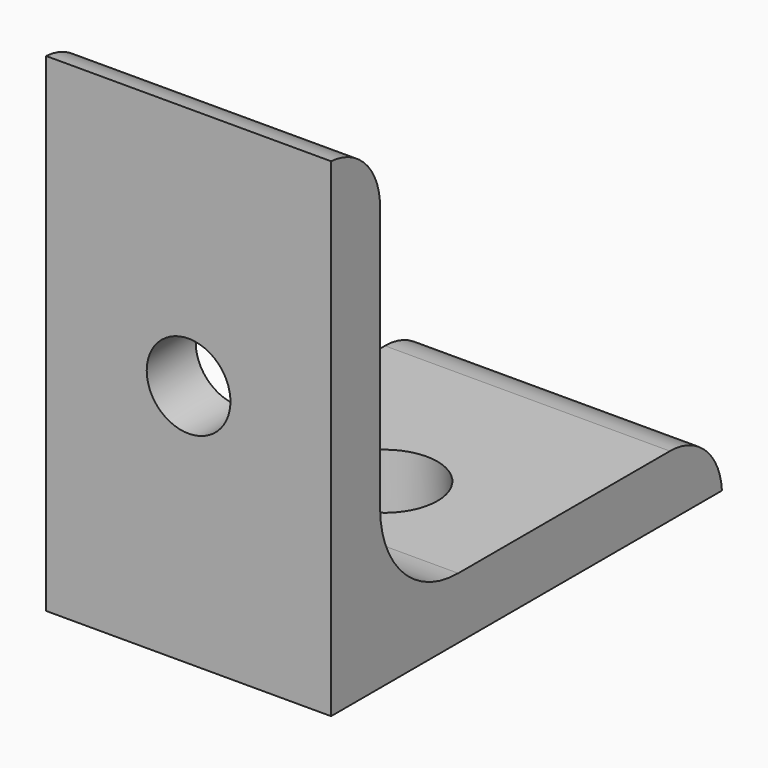
from build123d import *

# Parameters (mm, degrees)
F1_DEPTH    = 22.225
F2_R        = 7.62
F3_T1_DEPTH = 47.5792387778
F4_R        = 3.2639
F5_DEPTH    = 4.7762
F6_R        = 4.1656
F7_DEPTH    = 4.7762


# Not quite as in the source:
# - a fillet or chamfer that OpenCascade refuses, or shapes differently, is made with other operations: its cross-section is extruded or revolved along the edge and cut away or added


with BuildPart() as f1:
    # F0 (on Right) → F1 (new body)
    with BuildSketch(Plane.YZ):
        Polygon((0, 38.1), (0, 0), (38.1, 0), (38.1, 4.7752), (4.7752, 4.7752), (4.7752, 38.1), align=None)
    extrude(amount=-F1_DEPTH)

    # F2
    f2_edges = [f1.edges().sort_by_distance(p)[0] for p in [
        (-11.1125, 4.7752, 4.7752),
    ]]
    fillet(f2_edges, radius=F2_R)

    # F3: fillet of radius 5.08 on 2 edges, made by hand

    # F3_s2 → F3_t1 (cut)
    with BuildSketch(Plane.YZ.offset(-34.9021193889)):
        with BuildLine():
            ThreePointArc((4.7752, 33.0291522444), (3.3934958238, 36.5118247815), (0, 38.1))
            Line((0, 38.1), (4.7752, 38.1))
            Line((4.7752, 38.1), (4.7752, 33.0291522444))
        make_face()
        with BuildLine():
            ThreePointArc((33.0291522444, 4.7752), (36.5118247815, 3.3934958238), (38.1, 0))
            Line((38.1, 0), (38.1, 4.7752))
            Line((38.1, 4.7752), (33.0291522444, 4.7752))
        make_face()
    extrude(amount=F3_T1_DEPTH, mode=Mode.SUBTRACT)

    # F4 (on face) → F5 (cut, through all)
    with BuildSketch(Plane(origin=(0, 4.7752, 0), x_dir=(-1, 0, 0), z_dir=(0, 1, 0))):
        with Locations((11.1125, 19.05)):
            Circle(F4_R)
    extrude(amount=-F5_DEPTH, mode=Mode.SUBTRACT)

    # F6 (on face) → F7 (cut, through all)
    with BuildSketch(Plane.XY.offset(4.7752)):
        with Locations((-11.1125, 19.05)):
            Circle(F6_R)
    extrude(amount=-F7_DEPTH, mode=Mode.SUBTRACT)


solid = f1.part
